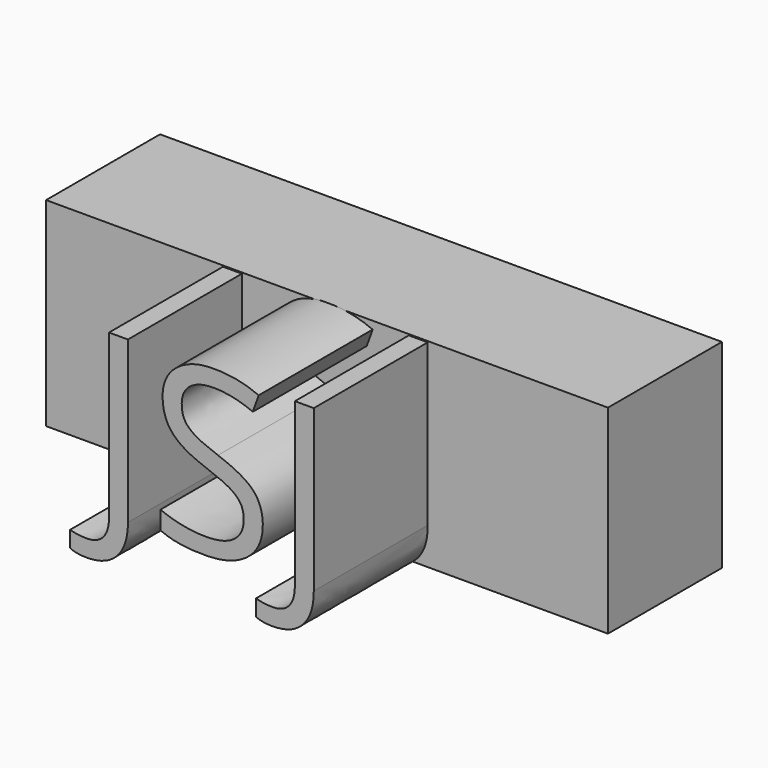
from build123d import *

# Parameters (mm, degrees)
F0_W         = 100.1968532801
F0_H         = 35.488307476
F1_DEPTH     = 25.4
F2_TEXT_SIZE = 40.616418442
F3_DEPTH     = 25.4


# Not quite as in the source:
# - Text() gives the source's letters only with a copy of the font that has no kerning and outlines rounded to 1/6400 em; it was checked with that copy


with BuildPart() as f1:
    # F0 (on Front) → F1 (new body)
    with BuildSketch(Plane.XZ):
        with Locations((50.09842664, 17.744153738)):
            Rectangle(F0_W, F0_H)
    extrude(amount=F1_DEPTH)

    # F2 (on face) → F3 (join)
    with BuildSketch(Plane.XZ.offset(25.4)):
        with Locations((27.7748359367, 6.2848287635)):
            Text('JSJ', F2_TEXT_SIZE, font='Open Sans', text_align=(TextAlign.LEFT, TextAlign.BOTTOM))
    extrude(amount=F3_DEPTH)


solid = f1.part
